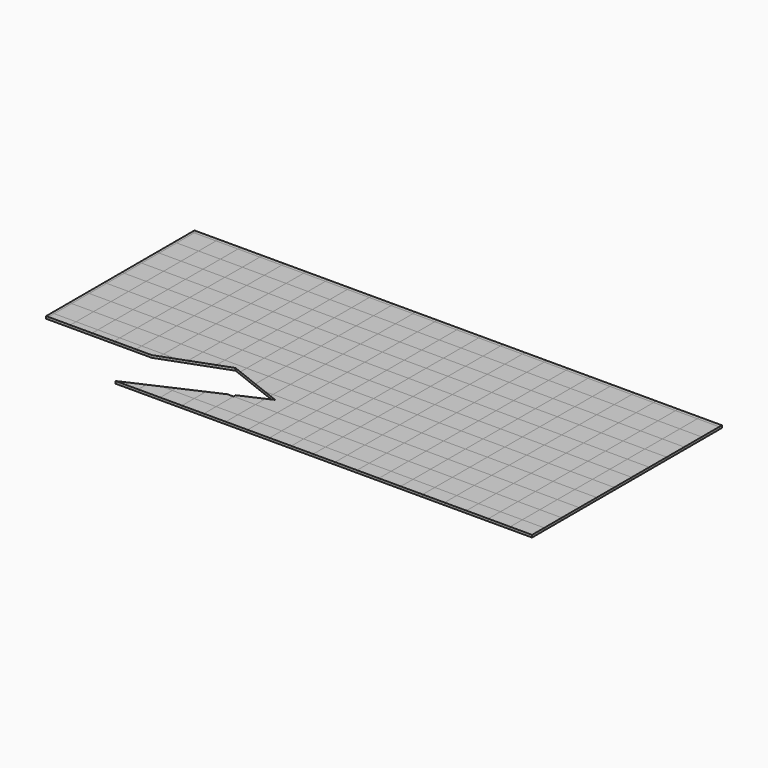
from build123d import *

# Parameters (mm, degrees)
F0_W     = 230
F0_H     = 35
F0_H_2   = 230
F0_H_3   = 160
F0_H_4   = 75
F0_W_2   = 25
F1_DEPTH = 25
F2_DEPTH = 25


with BuildPart() as f1:
    # F0 (on Top) → F1 (new body)
    with BuildSketch(Plane.XY):
        with Locations((2657.5, 1230)):
            Rectangle(F0_W, F0_H)
        with Locations((2427.5, 1097.5)):
            Rectangle(F0_W, F0_H_2)
        with Locations((2197.5, 867.5)):
            Rectangle(F0_W, F0_H_2)
        with Locations((1967.5, 637.5)):
            Rectangle(F0_W, F0_H_2)
        with Locations((1737.5, 407.5)):
            Rectangle(F0_W, F0_H_2)
        with Locations((1047.5, -282.5)):
            Rectangle(F0_W, F0_H_2)
        with Locations((817.5, -512.5)):
            Rectangle(F0_W, F0_H_2)
        with Locations((1507.5, 177.5)):
            Rectangle(F0_W, F0_H_2)
        with Locations((2657.5, 867.5)):
            Rectangle(F0_W, F0_H_2)
        with Locations((2427.5, 637.5)):
            Rectangle(F0_W, F0_H_2)
        with Locations((2197.5, 407.5)):
            Rectangle(F0_W, F0_H_2)
        with Locations((1967.5, 177.5)):
            Rectangle(F0_W, F0_H_2)
        with Locations((1737.5, -52.5)):
            Rectangle(F0_W, F0_H_2)
        with Locations((1507.5, -282.5)):
            Rectangle(F0_W, F0_H_2)
        with Locations((1277.5, -52.5)):
            Rectangle(F0_W, F0_H_2)
        with Locations((1277.5, -512.5)):
            Rectangle(F0_W, F0_H_2)
        with Locations((1737.5, -512.5)):
            Rectangle(F0_W, F0_H_2)
        with Locations((2197.5, -512.5)):
            Rectangle(F0_W, F0_H_2)
        with Locations((2657.5, -512.5)):
            Rectangle(F0_W, F0_H_2)
        with Locations((2427.5, -282.5)):
            Rectangle(F0_W, F0_H_2)
        with Locations((2197.5, -52.5)):
            Rectangle(F0_W, F0_H_2)
        with Locations((1967.5, -282.5)):
            Rectangle(F0_W, F0_H_2)
        with Locations((2427.5, 177.5)):
            Rectangle(F0_W, F0_H_2)
        with Locations((2657.5, 407.5)):
            Rectangle(F0_W, F0_H_2)
        with Locations((2657.5, -52.5)):
            Rectangle(F0_W, F0_H_2)
        with Locations((2427.5, -742.5)):
            Rectangle(F0_W, F0_H_2)
        with Locations((2197.5, -972.5)):
            Rectangle(F0_W, F0_H_2)
        with Locations((1967.5, -1167.5)):
            Rectangle(F0_W, F0_H_3)
        with Locations((2657.5, -972.5)):
            Rectangle(F0_W, F0_H_2)
        with Locations((2427.5, -1167.5)):
            Rectangle(F0_W, F0_H_3)
        with Locations((1967.5, -742.5)):
            Rectangle(F0_W, F0_H_2)
        with Locations((1737.5, -972.5)):
            Rectangle(F0_W, F0_H_2)
        with Locations((1507.5, -742.5)):
            Rectangle(F0_W, F0_H_2)
        with Locations((1277.5, -972.5)):
            Rectangle(F0_W, F0_H_2)
        with Locations((1047.5, -1167.5)):
            Rectangle(F0_W, F0_H_3)
        with Locations((1047.5, -742.5)):
            Rectangle(F0_W, F0_H_2)
        with Locations((817.5, -972.5)):
            Rectangle(F0_W, F0_H_2)
        with Locations((587.5, -1167.5)):
            Rectangle(F0_W, F0_H_3)
        with Locations((127.5, -1167.5)):
            Rectangle(F0_W, F0_H_3)
        with Locations((-332.5, -1167.5)):
            Rectangle(F0_W, F0_H_3)
        with Locations((-792.5, -1167.5)):
            Rectangle(F0_W, F0_H_3)
        with Locations((357.5, -972.5)):
            Rectangle(F0_W, F0_H_2)
        with Locations((587.5, -742.5)):
            Rectangle(F0_W, F0_H_2)
        with Locations((-102.5, -972.5)):
            Rectangle(F0_W, F0_H_2)
        with Locations((-562.5, -972.5)):
            Rectangle(F0_W, F0_H_2)
        Polygon((-1137.5, -1087.5), (-907.5, -1087.5), (-907.5, -932.3274866624), (-1137.5, -1036.022022707), align=None)
        Polygon((-1367.5, -1247.5), (-1137.5, -1247.5), (-1137.5, -1087.5), (-1251.6808935072, -1087.5), (-1367.5, -1139.7165587516), align=None)
        Polygon((-447.5, -857.5), (-217.5, -857.5), (-217.5, -627.5), (-447.5, -627.5), (-447.5, -661.8143741618), (-372.7013154673, -691.2157411411), (-447.5, -724.9384145732), align=None)
        with Locations((127.5, -742.5)):
            Rectangle(F0_W, F0_H_2)
        with Locations((357.5, -512.5)):
            Rectangle(F0_W, F0_H_2)
        with Locations((-102.5, -512.5)):
            Rectangle(F0_W, F0_H_2)
        Polygon((-534.797643326, -627.5), (-447.5, -627.5), (-447.5, -397.5), (-677.5, -397.5), (-677.5, -571.4075114274), align=None)
        with Locations((127.5, -282.5)):
            Rectangle(F0_W, F0_H_2)
        with Locations((587.5, -282.5)):
            Rectangle(F0_W, F0_H_2)
        with Locations((817.5, -52.5)):
            Rectangle(F0_W, F0_H_2)
        with Locations((1047.5, 177.5)):
            Rectangle(F0_W, F0_H_2)
        with Locations((1507.5, 637.5)):
            Rectangle(F0_W, F0_H_2)
        with Locations((1737.5, 867.5)):
            Rectangle(F0_W, F0_H_2)
        with Locations((1277.5, 407.5)):
            Rectangle(F0_W, F0_H_2)
        with Locations((1967.5, 1097.5)):
            Rectangle(F0_W, F0_H_2)
        with Locations((1507.5, 1097.5)):
            Rectangle(F0_W, F0_H_2)
        with Locations((1277.5, 867.5)):
            Rectangle(F0_W, F0_H_2)
        with Locations((1047.5, 637.5)):
            Rectangle(F0_W, F0_H_2)
        with Locations((817.5, 407.5)):
            Rectangle(F0_W, F0_H_2)
        with Locations((587.5, 177.5)):
            Rectangle(F0_W, F0_H_2)
        with Locations((357.5, -52.5)):
            Rectangle(F0_W, F0_H_2)
        with Locations((-332.5, -282.5)):
            Rectangle(F0_W, F0_H_2)
        with Locations((-102.5, -52.5)):
            Rectangle(F0_W, F0_H_2)
        with Locations((127.5, 177.5)):
            Rectangle(F0_W, F0_H_2)
        with Locations((587.5, 637.5)):
            Rectangle(F0_W, F0_H_2)
        with Locations((817.5, 867.5)):
            Rectangle(F0_W, F0_H_2)
        with Locations((1047.5, 1097.5)):
            Rectangle(F0_W, F0_H_2)
        with Locations((357.5, 407.5)):
            Rectangle(F0_W, F0_H_2)
        with Locations((587.5, 1097.5)):
            Rectangle(F0_W, F0_H_2)
        with Locations((357.5, 867.5)):
            Rectangle(F0_W, F0_H_2)
        with Locations((127.5, 637.5)):
            Rectangle(F0_W, F0_H_2)
        with Locations((-102.5, 407.5)):
            Rectangle(F0_W, F0_H_2)
        with Locations((-332.5, 177.5)):
            Rectangle(F0_W, F0_H_2)
        with Locations((-562.5, -52.5)):
            Rectangle(F0_W, F0_H_2)
        with Locations((-792.5, -282.5)):
            Rectangle(F0_W, F0_H_2)
        Polygon((-907.5, -481.0006486931), (-907.5, -397.5), (-1137.5, -397.5), (-1137.5, -508.8472179412), (-982.2986845327, -451.5992817137), align=None)
        Polygon((-1367.5, -593.6855796051), (-1367.5, -397.5), (-1597.5, -397.5), (-1597.5, -627.5), (-1459.1721697391, -627.5), align=None)
        with Locations((-1022.5, -52.5)):
            Rectangle(F0_W, F0_H_2)
        with Locations((-1252.5, -282.5)):
            Rectangle(F0_W, F0_H_2)
        with Locations((-792.5, 177.5)):
            Rectangle(F0_W, F0_H_2)
        with Locations((-562.5, 407.5)):
            Rectangle(F0_W, F0_H_2)
        with Locations((-332.5, 637.5)):
            Rectangle(F0_W, F0_H_2)
        with Locations((-102.5, 867.5)):
            Rectangle(F0_W, F0_H_2)
        with Locations((127.5, 1097.5)):
            Rectangle(F0_W, F0_H_2)
        with Locations((-332.5, 1097.5)):
            Rectangle(F0_W, F0_H_2)
        with Locations((-562.5, 867.5)):
            Rectangle(F0_W, F0_H_2)
        with Locations((-792.5, 637.5)):
            Rectangle(F0_W, F0_H_2)
        with Locations((-1022.5, 407.5)):
            Rectangle(F0_W, F0_H_2)
        with Locations((-1252.5, 177.5)):
            Rectangle(F0_W, F0_H_2)
        with Locations((-1482.5, -52.5)):
            Rectangle(F0_W, F0_H_2)
        with Locations((-1712.5, -282.5)):
            Rectangle(F0_W, F0_H_2)
        with Locations((-1942.5, -512.5)):
            Rectangle(F0_W, F0_H_2)
        with Locations((-2402.5, -512.5)):
            Rectangle(F0_W, F0_H_2)
        with Locations((-2172.5, -282.5)):
            Rectangle(F0_W, F0_H_2)
        with Locations((-1712.5, 177.5)):
            Rectangle(F0_W, F0_H_2)
        with Locations((-1482.5, 407.5)):
            Rectangle(F0_W, F0_H_2)
        with Locations((-1252.5, 637.5)):
            Rectangle(F0_W, F0_H_2)
        with Locations((-1022.5, 867.5)):
            Rectangle(F0_W, F0_H_2)
        with Locations((-792.5, 1097.5)):
            Rectangle(F0_W, F0_H_2)
        with Locations((-1942.5, -52.5)):
            Rectangle(F0_W, F0_H_2)
        with Locations((-1252.5, 1097.5)):
            Rectangle(F0_W, F0_H_2)
        with Locations((-1712.5, 1097.5)):
            Rectangle(F0_W, F0_H_2)
        with Locations((-2172.5, 1097.5)):
            Rectangle(F0_W, F0_H_2)
        with Locations((-2632.5, 1097.5)):
            Rectangle(F0_W, F0_H_2)
        with Locations((-1942.5, 867.5)):
            Rectangle(F0_W, F0_H_2)
        with Locations((-1482.5, 867.5)):
            Rectangle(F0_W, F0_H_2)
        with Locations((-2402.5, 867.5)):
            Rectangle(F0_W, F0_H_2)
        with Locations((-2172.5, 637.5)):
            Rectangle(F0_W, F0_H_2)
        with Locations((-1712.5, 637.5)):
            Rectangle(F0_W, F0_H_2)
        with Locations((-2632.5, 637.5)):
            Rectangle(F0_W, F0_H_2)
        with Locations((-1942.5, 407.5)):
            Rectangle(F0_W, F0_H_2)
        with Locations((-2172.5, 177.5)):
            Rectangle(F0_W, F0_H_2)
        with Locations((-2402.5, 407.5)):
            Rectangle(F0_W, F0_H_2)
        with Locations((-2632.5, 177.5)):
            Rectangle(F0_W, F0_H_2)
        with Locations((-2402.5, -52.5)):
            Rectangle(F0_W, F0_H_2)
        with Locations((-2632.5, -282.5)):
            Rectangle(F0_W, F0_H_2)
        with Locations((-2172.5, -665)):
            Rectangle(F0_W, F0_H_4)
        Polygon((-1597.5, -678.5239412689), (-1597.5, -627.5), (-1827.5, -627.5), (-1827.5, -702.5), (-1662.5, -702.5), align=None)
        with Locations((-2632.5, -665)):
            Rectangle(F0_W, F0_H_4)
        with Locations((-2760, -512.5)):
            Rectangle(F0_W_2, F0_H_2)
        with Locations((-2760, -52.5)):
            Rectangle(F0_W_2, F0_H_2)
        with Locations((-2760, 407.5)):
            Rectangle(F0_W_2, F0_H_2)
        with Locations((-2760, 867.5)):
            Rectangle(F0_W_2, F0_H_2)
        Polygon((-2772.5, 1212.5), (-2747.5, 1212.5), (-2747.5, 1247.5), (-2772.5, 1247.5), (-2772.5, 1217.5), align=None)
        with Locations((-2402.5, 1230)):
            Rectangle(F0_W, F0_H)
        with Locations((-1942.5, 1230)):
            Rectangle(F0_W, F0_H)
        with Locations((-1022.5, 1230)):
            Rectangle(F0_W, F0_H)
        with Locations((-1482.5, 1230)):
            Rectangle(F0_W, F0_H)
        with Locations((-562.5, 1230)):
            Rectangle(F0_W, F0_H)
        with Locations((-102.5, 1230)):
            Rectangle(F0_W, F0_H)
        with Locations((357.5, 1230)):
            Rectangle(F0_W, F0_H)
        with Locations((817.5, 1230)):
            Rectangle(F0_W, F0_H)
        with Locations((1277.5, 1230)):
            Rectangle(F0_W, F0_H)
        with Locations((1737.5, 1230)):
            Rectangle(F0_W, F0_H)
        with Locations((2197.5, 1230)):
            Rectangle(F0_W, F0_H)
        with Locations((1507.5, -1167.5)):
            Rectangle(F0_W, F0_H_3)
    extrude(amount=F1_DEPTH)


with BuildPart() as f2:
    # F0 (on Top) → F2 (new body)
    with BuildSketch(Plane.XY):
        with Locations((2657.5, -1167.5)):
            Rectangle(F0_W, F0_H_3)
        with Locations((2427.5, -972.5)):
            Rectangle(F0_W, F0_H_2)
        with Locations((2197.5, -1167.5)):
            Rectangle(F0_W, F0_H_3)
        with Locations((2657.5, -742.5)):
            Rectangle(F0_W, F0_H_2)
        with Locations((2197.5, -742.5)):
            Rectangle(F0_W, F0_H_2)
        with Locations((2427.5, -512.5)):
            Rectangle(F0_W, F0_H_2)
        with Locations((2657.5, -282.5)):
            Rectangle(F0_W, F0_H_2)
        with Locations((1967.5, -972.5)):
            Rectangle(F0_W, F0_H_2)
        with Locations((1737.5, -1167.5)):
            Rectangle(F0_W, F0_H_3)
        with Locations((1737.5, -742.5)):
            Rectangle(F0_W, F0_H_2)
        with Locations((1967.5, -512.5)):
            Rectangle(F0_W, F0_H_2)
        with Locations((2427.5, -52.5)):
            Rectangle(F0_W, F0_H_2)
        with Locations((2197.5, -282.5)):
            Rectangle(F0_W, F0_H_2)
        with Locations((2657.5, 177.5)):
            Rectangle(F0_W, F0_H_2)
        with Locations((2657.5, 637.5)):
            Rectangle(F0_W, F0_H_2)
        with Locations((2427.5, 407.5)):
            Rectangle(F0_W, F0_H_2)
        with Locations((2197.5, 177.5)):
            Rectangle(F0_W, F0_H_2)
        with Locations((1967.5, -52.5)):
            Rectangle(F0_W, F0_H_2)
        with Locations((1737.5, -282.5)):
            Rectangle(F0_W, F0_H_2)
        with Locations((1507.5, -512.5)):
            Rectangle(F0_W, F0_H_2)
        with Locations((1277.5, -742.5)):
            Rectangle(F0_W, F0_H_2)
        with Locations((1047.5, -972.5)):
            Rectangle(F0_W, F0_H_2)
        with Locations((1277.5, -1167.5)):
            Rectangle(F0_W, F0_H_3)
        with Locations((1507.5, -972.5)):
            Rectangle(F0_W, F0_H_2)
        with Locations((2657.5, 1097.5)):
            Rectangle(F0_W, F0_H_2)
        with Locations((2427.5, 867.5)):
            Rectangle(F0_W, F0_H_2)
        with Locations((2197.5, 637.5)):
            Rectangle(F0_W, F0_H_2)
        with Locations((1967.5, 407.5)):
            Rectangle(F0_W, F0_H_2)
        with Locations((1737.5, 177.5)):
            Rectangle(F0_W, F0_H_2)
        with Locations((1507.5, -52.5)):
            Rectangle(F0_W, F0_H_2)
        with Locations((1277.5, -282.5)):
            Rectangle(F0_W, F0_H_2)
        with Locations((1047.5, -512.5)):
            Rectangle(F0_W, F0_H_2)
        with Locations((587.5, -972.5)):
            Rectangle(F0_W, F0_H_2)
        with Locations((357.5, -1167.5)):
            Rectangle(F0_W, F0_H_3)
        with Locations((817.5, -1167.5)):
            Rectangle(F0_W, F0_H_3)
        with Locations((817.5, -742.5)):
            Rectangle(F0_W, F0_H_2)
        with Locations((817.5, -282.5)):
            Rectangle(F0_W, F0_H_2)
        with Locations((2197.5, 1097.5)):
            Rectangle(F0_W, F0_H_2)
        with Locations((1967.5, 867.5)):
            Rectangle(F0_W, F0_H_2)
        with Locations((1277.5, 177.5)):
            Rectangle(F0_W, F0_H_2)
        with Locations((1507.5, 407.5)):
            Rectangle(F0_W, F0_H_2)
        with Locations((1737.5, 637.5)):
            Rectangle(F0_W, F0_H_2)
        with Locations((1047.5, -52.5)):
            Rectangle(F0_W, F0_H_2)
        with Locations((587.5, -512.5)):
            Rectangle(F0_W, F0_H_2)
        with Locations((357.5, -742.5)):
            Rectangle(F0_W, F0_H_2)
        with Locations((127.5, -972.5)):
            Rectangle(F0_W, F0_H_2)
        with Locations((-102.5, -1167.5)):
            Rectangle(F0_W, F0_H_3)
        with Locations((-562.5, -1167.5)):
            Rectangle(F0_W, F0_H_3)
        with Locations((-1022.5, -1167.5)):
            Rectangle(F0_W, F0_H_3)
        Polygon((-1606.5694093704, -1247.5), (-1367.5, -1247.5), (-1367.5, -1139.7165587516), align=None)
        Polygon((-907.5, -1087.5), (-677.5, -1087.5), (-677.5, -857.5), (-741.5286519538, -857.5), (-907.5, -932.3274866624), align=None)
        with Locations((-332.5, -972.5)):
            Rectangle(F0_W, F0_H_2)
        Polygon((-677.5, -857.5), (-447.5, -857.5), (-447.5, -724.9384145732), (-677.5, -828.6329506178), align=None)
        with Locations((-102.5, -742.5)):
            Rectangle(F0_W, F0_H_2)
        with Locations((127.5, -512.5)):
            Rectangle(F0_W, F0_H_2)
        with Locations((-332.5, -512.5)):
            Rectangle(F0_W, F0_H_2)
        with Locations((-102.5, -282.5)):
            Rectangle(F0_W, F0_H_2)
        with Locations((357.5, -282.5)):
            Rectangle(F0_W, F0_H_2)
        with Locations((127.5, -52.5)):
            Rectangle(F0_W, F0_H_2)
        with Locations((817.5, 177.5)):
            Rectangle(F0_W, F0_H_2)
        with Locations((357.5, 177.5)):
            Rectangle(F0_W, F0_H_2)
        with Locations((1047.5, 407.5)):
            Rectangle(F0_W, F0_H_2)
        with Locations((587.5, -52.5)):
            Rectangle(F0_W, F0_H_2)
        with Locations((1277.5, 637.5)):
            Rectangle(F0_W, F0_H_2)
        with Locations((1507.5, 867.5)):
            Rectangle(F0_W, F0_H_2)
        with Locations((1737.5, 1097.5)):
            Rectangle(F0_W, F0_H_2)
        with Locations((1277.5, 1097.5)):
            Rectangle(F0_W, F0_H_2)
        with Locations((1047.5, 867.5)):
            Rectangle(F0_W, F0_H_2)
        with Locations((817.5, 637.5)):
            Rectangle(F0_W, F0_H_2)
        with Locations((587.5, 407.5)):
            Rectangle(F0_W, F0_H_2)
        with Locations((817.5, 1097.5)):
            Rectangle(F0_W, F0_H_2)
        with Locations((587.5, 867.5)):
            Rectangle(F0_W, F0_H_2)
        with Locations((357.5, 637.5)):
            Rectangle(F0_W, F0_H_2)
        with Locations((127.5, 407.5)):
            Rectangle(F0_W, F0_H_2)
        with Locations((-102.5, 177.5)):
            Rectangle(F0_W, F0_H_2)
        with Locations((-332.5, -52.5)):
            Rectangle(F0_W, F0_H_2)
        with Locations((-562.5, -282.5)):
            Rectangle(F0_W, F0_H_2)
        Polygon((-677.5, -571.4075114274), (-677.5, -397.5), (-907.5, -397.5), (-907.5, -481.0006486931), align=None)
        with Locations((-1942.5, -282.5)):
            Rectangle(F0_W, F0_H_2)
        Polygon((-1137.5, -508.8472179412), (-1137.5, -397.5), (-1367.5, -397.5), (-1367.5, -593.6855796051), align=None)
        with Locations((-1712.5, -512.5)):
            Rectangle(F0_W, F0_H_2)
        with Locations((-2172.5, -512.5)):
            Rectangle(F0_W, F0_H_2)
        with Locations((-2632.5, -512.5)):
            Rectangle(F0_W, F0_H_2)
        with Locations((-2402.5, -282.5)):
            Rectangle(F0_W, F0_H_2)
        with Locations((-1482.5, -282.5)):
            Rectangle(F0_W, F0_H_2)
        with Locations((-1022.5, -282.5)):
            Rectangle(F0_W, F0_H_2)
        with Locations((-792.5, -52.5)):
            Rectangle(F0_W, F0_H_2)
        with Locations((-562.5, 177.5)):
            Rectangle(F0_W, F0_H_2)
        with Locations((-332.5, 407.5)):
            Rectangle(F0_W, F0_H_2)
        with Locations((-102.5, 637.5)):
            Rectangle(F0_W, F0_H_2)
        with Locations((127.5, 867.5)):
            Rectangle(F0_W, F0_H_2)
        with Locations((357.5, 1097.5)):
            Rectangle(F0_W, F0_H_2)
        with Locations((-102.5, 1097.5)):
            Rectangle(F0_W, F0_H_2)
        with Locations((-332.5, 867.5)):
            Rectangle(F0_W, F0_H_2)
        with Locations((-562.5, 637.5)):
            Rectangle(F0_W, F0_H_2)
        with Locations((-792.5, 407.5)):
            Rectangle(F0_W, F0_H_2)
        with Locations((-1252.5, -52.5)):
            Rectangle(F0_W, F0_H_2)
        with Locations((-1712.5, -52.5)):
            Rectangle(F0_W, F0_H_2)
        with Locations((-1482.5, 177.5)):
            Rectangle(F0_W, F0_H_2)
        with Locations((-1022.5, 177.5)):
            Rectangle(F0_W, F0_H_2)
        with Locations((-1252.5, 407.5)):
            Rectangle(F0_W, F0_H_2)
        with Locations((-1022.5, 637.5)):
            Rectangle(F0_W, F0_H_2)
        with Locations((-792.5, 867.5)):
            Rectangle(F0_W, F0_H_2)
        with Locations((-562.5, 1097.5)):
            Rectangle(F0_W, F0_H_2)
        with Locations((-1022.5, 1097.5)):
            Rectangle(F0_W, F0_H_2)
        with Locations((-1252.5, 867.5)):
            Rectangle(F0_W, F0_H_2)
        with Locations((-1482.5, 637.5)):
            Rectangle(F0_W, F0_H_2)
        with Locations((-1712.5, 407.5)):
            Rectangle(F0_W, F0_H_2)
        with Locations((-1942.5, 177.5)):
            Rectangle(F0_W, F0_H_2)
        with Locations((-2172.5, -52.5)):
            Rectangle(F0_W, F0_H_2)
        with Locations((-2402.5, 177.5)):
            Rectangle(F0_W, F0_H_2)
        with Locations((-2632.5, -52.5)):
            Rectangle(F0_W, F0_H_2)
        with Locations((-2172.5, 407.5)):
            Rectangle(F0_W, F0_H_2)
        with Locations((-2632.5, 407.5)):
            Rectangle(F0_W, F0_H_2)
        with Locations((-2402.5, 637.5)):
            Rectangle(F0_W, F0_H_2)
        with Locations((-1942.5, 637.5)):
            Rectangle(F0_W, F0_H_2)
        with Locations((-2172.5, 867.5)):
            Rectangle(F0_W, F0_H_2)
        with Locations((-2632.5, 867.5)):
            Rectangle(F0_W, F0_H_2)
        with Locations((-2402.5, 1097.5)):
            Rectangle(F0_W, F0_H_2)
        with Locations((-1942.5, 1097.5)):
            Rectangle(F0_W, F0_H_2)
        with Locations((-1712.5, 867.5)):
            Rectangle(F0_W, F0_H_2)
        with Locations((-1482.5, 1097.5)):
            Rectangle(F0_W, F0_H_2)
        with Locations((2427.5, 1230)):
            Rectangle(F0_W, F0_H)
        with Locations((1967.5, 1230)):
            Rectangle(F0_W, F0_H)
        with Locations((1507.5, 1230)):
            Rectangle(F0_W, F0_H)
        with Locations((1047.5, 1230)):
            Rectangle(F0_W, F0_H)
        with Locations((587.5, 1230)):
            Rectangle(F0_W, F0_H)
        with Locations((127.5, 1230)):
            Rectangle(F0_W, F0_H)
        with Locations((-332.5, 1230)):
            Rectangle(F0_W, F0_H)
        with Locations((-792.5, 1230)):
            Rectangle(F0_W, F0_H)
        with Locations((-1252.5, 1230)):
            Rectangle(F0_W, F0_H)
        with Locations((-1712.5, 1230)):
            Rectangle(F0_W, F0_H)
        with Locations((-2172.5, 1230)):
            Rectangle(F0_W, F0_H)
        with Locations((-2632.5, 1230)):
            Rectangle(F0_W, F0_H)
        with Locations((-2760, 1097.5)):
            Rectangle(F0_W_2, F0_H_2)
        with Locations((-2760, 637.5)):
            Rectangle(F0_W_2, F0_H_2)
        with Locations((-2760, 177.5)):
            Rectangle(F0_W_2, F0_H_2)
        with Locations((-2760, -282.5)):
            Rectangle(F0_W_2, F0_H_2)
        with Locations((-2760, -665)):
            Rectangle(F0_W_2, F0_H_4)
        with Locations((-2402.5, -665)):
            Rectangle(F0_W, F0_H_4)
        with Locations((-1942.5, -665)):
            Rectangle(F0_W, F0_H_4)
        Polygon((-1459.1721697391, -627.5), (-1597.5, -627.5), (-1597.5, -678.5239412689), align=None)
        Polygon((-1251.6808935072, -1087.5), (-1137.5, -1087.5), (-1137.5, -1036.022022707), align=None)
        Polygon((-447.5, -661.8143741618), (-447.5, -627.5), (-534.797643326, -627.5), align=None)
    extrude(amount=F2_DEPTH)


solid = Compound([f1.part, f2.part])
